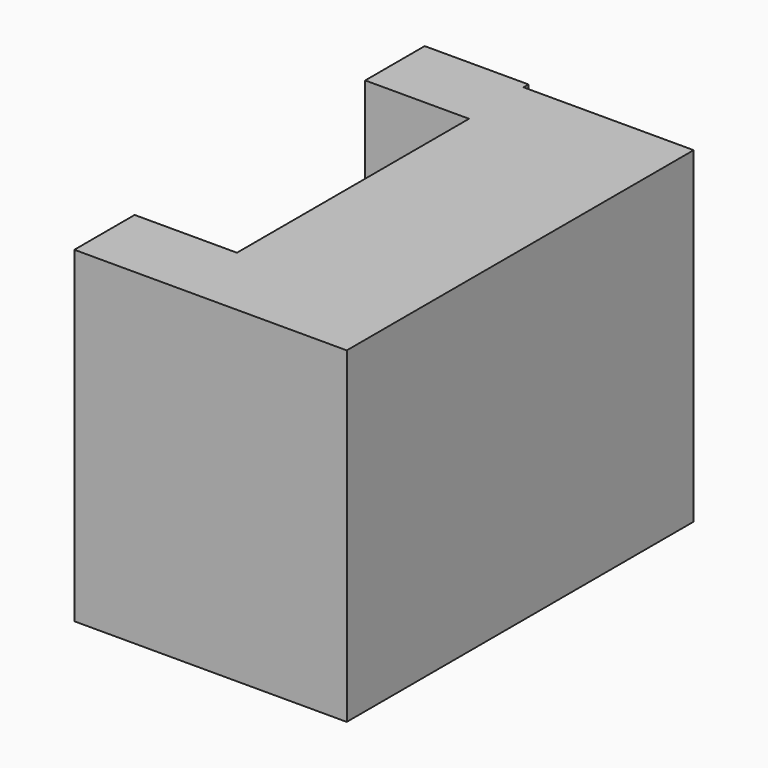
from build123d import *

# Parameters (mm, degrees)
F2_W     = 5.9578604996
F2_H     = 4.390229471
F3_DEPTH = 19.05


# Not quite as in the source:
# - the program builds the solid bodies; features that only make, move or delete a surface that nothing else refers to are left out


with BuildPart() as f3:
    # F2 (on Top) → F3 (new body)
    with BuildSketch(Plane.XY):
        Polygon((48.7568192184, 33.4314107895), (38.8487800956, 33.4314107895), (38.8487800956, 29.4627081603), (38.8487800956, 12.5663736835), (38.8487800956, 8.1761442125), (48.7568192184, 8.1761442125), align=None)
        Polygon((38.8487800956, 29.4627081603), (38.8487800956, 33.4314107895), (38.8487800956, 33.7930396199), (32.8023135662, 33.7930396199), (32.8023135662, 29.4627081603), align=None)
        with Locations((35.8698498458, 10.371258948)):
            Rectangle(F2_W, F2_H)
    extrude(amount=F3_DEPTH)


solid = f3.part
